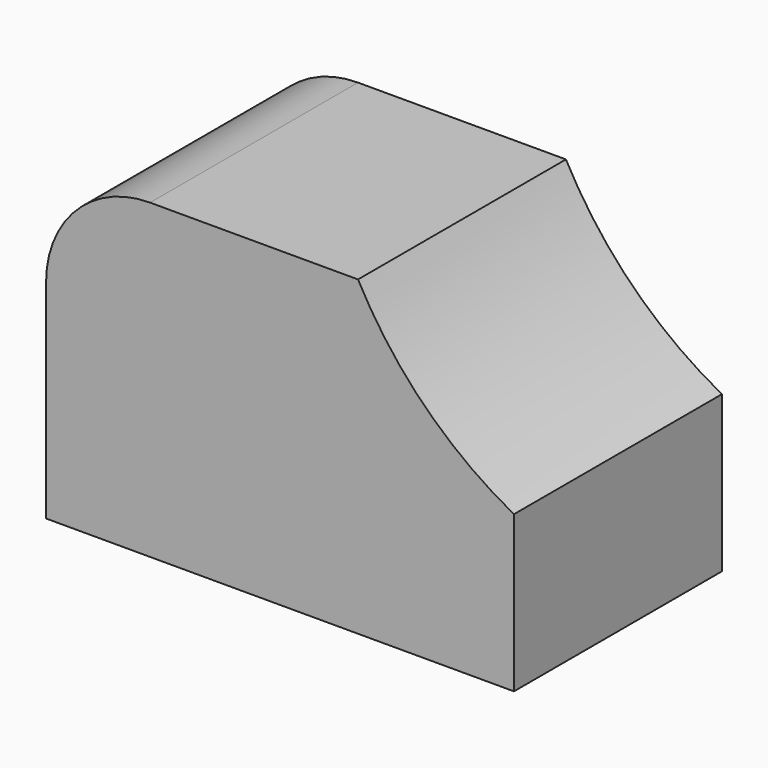
from build123d import *

# Parameters (mm, degrees)
F0_W     = 57.15
F0_H     = 38.1
F1_DEPTH = 31.75
F3_DEPTH = 31.75
F5_DEPTH = 31.75


# Not quite as in the source:
# - a length typed as a fraction of an inch, garbled in the dataset ("3 / 203.2 mm" for 3/8 in), is restored
# - a feature names something its author has since deleted; it is built from what else it names


with BuildPart() as f1:
    # F0 (on Front) → F1 (new body)
    with BuildSketch(Plane.XZ):
        with Locations((28.575, 19.05)):
            Rectangle(F0_W, F0_H)
    extrude(amount=F1_DEPTH)

    # F2 (on face) → F3 (cut)
    with BuildSketch(Plane.XZ.offset(31.75)):
        with BuildLine():
            Line((57.15, 38.1), (38.1, 38.1))
            ThreePointArc((38.1, 38.1), (46.2145934678, 27.1645934678), (57.15, 19.05))
            Line((57.15, 19.05), (57.15, 38.1))
        make_face()
    extrude(amount=-F3_DEPTH, mode=Mode.SUBTRACT)

    # F4 (on face) → F5 (cut)
    with BuildSketch(Plane.XZ.offset(31.75)):
        with BuildLine():
            Line((0, 38.1), (0, 25.4))
            ThreePointArc((0, 25.4), (3.7197438789, 34.3802561211), (12.7, 38.1))
            Line((12.7, 38.1), (0, 38.1))
        make_face()
    extrude(amount=-F5_DEPTH, mode=Mode.SUBTRACT)


solid = f1.part
